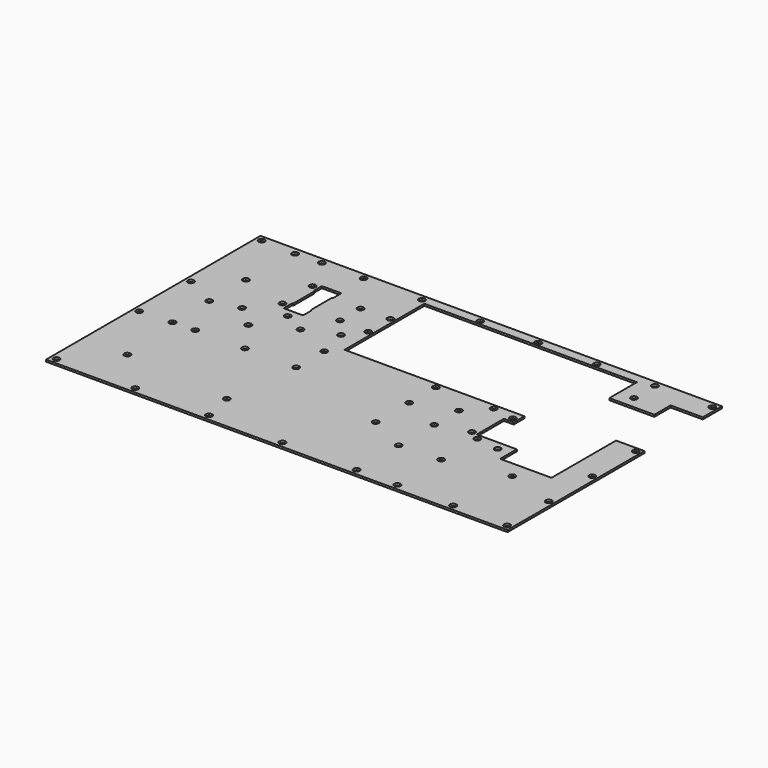
from build123d import *

# Parameters (mm, degrees)
F0_R     = 1.6
F1_DEPTH = 1


# Not quite as in the source:
# - ends of sketch curves that miss each other by under 0.0002 mm in the source are joined


with BuildPart() as f1:
    # F0 (on Top) → F1 (new body)
    with BuildSketch(Plane.XY):
        Polygon((102.2, 56.7), (113.5, 56.7), (118.8, 56.7), (118.8, 69), (-118.8, 69), (-118.8, -69), (118.8, -69), (118.8, 19.1), (118.7999, 19.1001), (113.553, 19.1001), (104.2105, 19.1005), (104.2, -22.45), (88.8825, -22.45), (77.8, -22.45), (77.8, -11.8), (57.15, -11.8), (57.15, 5.75), (62.2, 5.75), (62.2, 12.6), (37.3752, 12.5999), (-30.4, 12.6), (-30.4, 64), (37.3639, 64), (61.18, 64), (78.995, 64), (79.01, 64), (79.0100016935, 63.9849983065), (79.012, 46.283), (88.0852, 46.283), (102.2, 46.282), align=None)
        with Locations((-115.8, -66)):
            Circle(F0_R, mode=Mode.SUBTRACT)
        with Locations((-75.3, -66)):
            Circle(F0_R, mode=Mode.SUBTRACT)
        with Locations((-96.002, -45.2007)):
            Circle(F0_R, mode=Mode.SUBTRACT)
        with Locations((-37.3, -66)):
            Circle(F0_R, mode=Mode.SUBTRACT)
        with Locations((-40.7, -50.30003)):
            Circle(F0_R, mode=Mode.SUBTRACT)
        with Locations((-115.8, -12.8)):
            Circle(F0_R, mode=Mode.SUBTRACT)
        with Locations((-99.4, -11.9)):
            Circle(F0_R, mode=Mode.SUBTRACT)
        with Locations((-87.9916, -11.4944)):
            Circle(F0_R, mode=Mode.SUBTRACT)
        with Locations((-62.3953, -11.5044)):
            Circle(F0_R, mode=Mode.SUBTRACT)
        with Locations((-35.9953, -11.5044)):
            Circle(F0_R, mode=Mode.SUBTRACT)
        with Locations((0.5, -66)):
            Circle(F0_R, mode=Mode.SUBTRACT)
        with Locations((38.7, -66)):
            Circle(F0_R, mode=Mode.SUBTRACT)
        with Locations((38.6047, -38.8044)):
            Circle(F0_R, mode=Mode.SUBTRACT)
        with Locations((59.7, -66)):
            Circle(F0_R, mode=Mode.SUBTRACT)
        with Locations((88.4, -66)):
            Circle(F0_R, mode=Mode.SUBTRACT)
        with Locations((116.2, -66)):
            Circle(F0_R, mode=Mode.SUBTRACT)
        with Locations((59.6946, -37.8013)):
            Circle(F0_R, mode=Mode.SUBTRACT)
        with Locations((116.2, -39.2)):
            Circle(F0_R, mode=Mode.SUBTRACT)
        with Locations((18.7, -28.7)):
            Circle(F0_R, mode=Mode.SUBTRACT)
        with Locations((18.7, -7.2)):
            Circle(F0_R, mode=Mode.SUBTRACT)
        with Locations((38.6, -15.9)):
            Circle(F0_R, mode=Mode.SUBTRACT)
        with Locations((54.3, -11.30003)):
            Circle(F0_R, mode=Mode.SUBTRACT)
        with Locations((38.5947, -0.0044)):
            Circle(F0_R, mode=Mode.SUBTRACT)
        with Locations((91, -31.2)):
            Circle(F0_R, mode=Mode.SUBTRACT)
        with Locations((59.7, -14.6)):
            Circle(F0_R, mode=Mode.SUBTRACT)
        with Locations((71.6, -16.3)):
            Circle(F0_R, mode=Mode.SUBTRACT)
        with Locations((116.2, -11.2)):
            Circle(F0_R, mode=Mode.SUBTRACT)
        with Locations((-99.392, 11.7993)):
            Circle(F0_R, mode=Mode.SUBTRACT)
        with Locations((-74.0947, 5.3044)):
            Circle(F0_R, mode=Mode.SUBTRACT)
        with Locations((-85.3, 15.3)):
            Circle(F0_R, mode=Mode.SUBTRACT)
        with Locations((-115.8, 20.5)):
            Circle(F0_R, mode=Mode.SUBTRACT)
        with Locations((-66.6053, 21.28557)):
            Circle(F0_R, mode=Mode.SUBTRACT)
        with Locations((-75.0953, 28.4956)):
            Circle(F0_R, mode=Mode.SUBTRACT)
        with Locations((-35.9953, 6.4956)):
            Circle(F0_R, mode=Mode.SUBTRACT)
        with Locations((-55.2953, 15.3056)):
            Circle(F0_R, mode=Mode.SUBTRACT)
        with Locations((-39.5853, 21.8056)):
            Circle(F0_R, mode=Mode.SUBTRACT)
        with Locations((-47.8, 31.4)):
            Circle(F0_R, mode=Mode.SUBTRACT)
        with Locations((-32.8, 30.8)):
            Circle(F0_R, mode=Mode.SUBTRACT)
        with Locations((-99.392, 35.3993)):
            Circle(F0_R, mode=Mode.SUBTRACT)
        with BuildLine():
            ThreePointArc((-71.6712000014, 25.5657995631), (-72.0236133171, 25.7129538657), (-72.1690001854, 26.0661000003))
            Line((-72.1690001854, 26.0661000003), (-72.169, 30.6661))
            ThreePointArc((-72.169, 30.6661), (-72.022760123, 31.017660123), (-71.6711999992, 31.1638997499))
            Line((-71.6711999992, 31.1638997499), (-71.6712, 44.6361))
            ThreePointArc((-71.6712, 44.6361), (-72.022760123, 44.782339877), (-72.1689997499, 45.1339000008))
            Line((-72.1689997499, 45.1339000008), (-72.169, 49.7339))
            ThreePointArc((-72.169, 49.7339), (-72.0236133171, 50.0870461343), (-71.6712000014, 50.2342004369))
            Line((-71.6712000014, 50.2342004369), (-62.6288, 50.2342))
            ThreePointArc((-62.6288, 50.2342), (-62.2763866829, 50.0870461343), (-62.1309998146, 49.7338999997))
            Line((-62.1309998146, 49.7338999997), (-62.131, 45.1339))
            ThreePointArc((-62.131, 45.1339), (-62.277239877, 44.782339877), (-62.6288000008, 44.6361002501))
            Line((-62.6288000008, 44.6361002501), (-62.6288, 31.1639))
            ThreePointArc((-62.6288, 31.1639), (-62.277239877, 31.017660123), (-62.1310002501, 30.6660999992))
            Line((-62.1310002501, 30.6660999992), (-62.131, 26.0661))
            ThreePointArc((-62.131, 26.0661), (-62.2763866829, 25.7129538657), (-62.6287999986, 25.5657995631))
            Line((-62.6287999986, 25.5657995631), (-71.6712000014, 25.5657995631))
        make_face(mode=Mode.SUBTRACT)
        with Locations((-75.0953, 47.9056)):
            Circle(F0_R, mode=Mode.SUBTRACT)
        with Locations((-115.8, 66)):
            Circle(F0_R, mode=Mode.SUBTRACT)
        with Locations((-98.1, 65.4)):
            Circle(F0_R, mode=Mode.SUBTRACT)
        with Locations((-84.8, 66)):
            Circle(F0_R, mode=Mode.SUBTRACT)
        with Locations((-63.3, 66)):
            Circle(F0_R, mode=Mode.SUBTRACT)
        with Locations((-47.7953, 44.6956)):
            Circle(F0_R, mode=Mode.SUBTRACT)
        with Locations((-32.8, 45.1)):
            Circle(F0_R, mode=Mode.SUBTRACT)
        with Locations((-33.3, 66)):
            Circle(F0_R, mode=Mode.SUBTRACT)
        with Locations((-3.3, 66)):
            Circle(F0_R, mode=Mode.SUBTRACT)
        with Locations((18.7, 10)):
            Circle(F0_R, mode=Mode.SUBTRACT)
        with Locations((48.3948, 10.0954)):
            Circle(F0_R, mode=Mode.SUBTRACT)
        with Locations((59.698, 8.2993)):
            Circle(F0_R, mode=Mode.SUBTRACT)
        with Locations((116.2, 16.8)):
            Circle(F0_R, mode=Mode.SUBTRACT)
        with BuildLine():
            ThreePointArc((26.5840005, 64.4042105039), (24.868001, 66), (26.5840005, 67.5957894961))
            ThreePointArc((26.5840005, 67.5957894961), (27.7895872613, 67.1716653106), (28.3, 66))
            ThreePointArc((28.3, 66), (27.7895872613, 64.8283346894), (26.5840005, 64.4042105039))
        make_face(mode=Mode.SUBTRACT)
        with Locations((56.7, 66)):
            Circle(F0_R, mode=Mode.SUBTRACT)
        with Locations((86.7, 52.5)):
            Circle(F0_R, mode=Mode.SUBTRACT)
        with Locations((86.7, 66)):
            Circle(F0_R, mode=Mode.SUBTRACT)
        with Locations((116.2, 66)):
            Circle(F0_R, mode=Mode.SUBTRACT)
    extrude(amount=F1_DEPTH)


solid = f1.part
